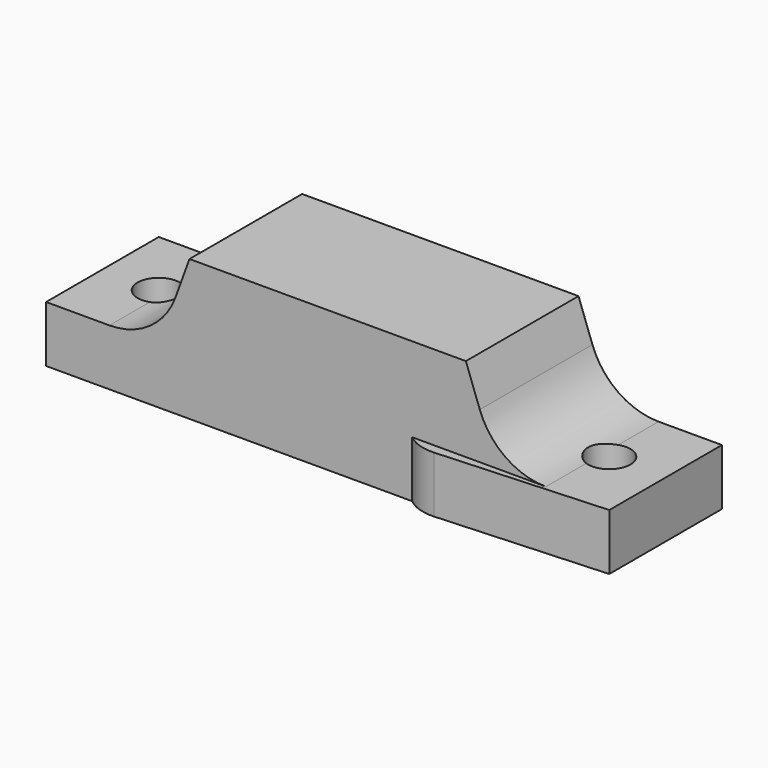
from build123d import *

# Parameters (mm, degrees)
F1_DEPTH    = 5
F2_R        = 5
F3_R        = 1.5
F4_DEPTH    = 25
F6_DEPTH    = 4
F7_T1_DEPTH = 14.4192067173


# Not quite as in the source:
# - a fillet or chamfer that OpenCascade refuses, or shapes differently, is made with other operations: its cross-section is extruded or revolved along the edge and cut away or added


with BuildPart() as f1:
    # F0 (on Front) → F1 (new body, symmetric)
    with BuildSketch(Plane.XZ):
        Polygon((0, 4), (0, 0), (40, 0), (40, 4), (32, 4), (29.8161785944, 10), (10.1838214056, 10), (8, 4), align=None)
    extrude(amount=F1_DEPTH, both=True)

    # F2
    f2_edges = [f1.edges().sort_by_distance(p)[0] for p in [
        (32, 0, 4),
        (8, 0, 4),
    ]]
    fillet(f2_edges, radius=F2_R)

    # F3 (on Top) → F4 (cut)
    with BuildSketch(Plane.XY):
        with Locations((4, 0)):
            Circle(F3_R)
        with Locations((36, 0)):
            Circle(F3_R)
    extrude(amount=F4_DEPTH, mode=Mode.SUBTRACT)

    # F5 (on Top) → F6 (join)
    with BuildSketch(Plane.XY):
        Polygon((26, -5.8), (40, -5), (26, -5), align=None)
    extrude(amount=F6_DEPTH)

    # F7: fillet of radius 3 on 1 edges, made by hand

    # F7_s2 → F7_t1 (cut)
    with BuildSketch(Plane.XY.offset(-5.2096033586)):
        with BuildLine():
            ThreePointArc((26, -5), (26.9758794109, -5.5370959816), (28.0804474628, -5.6811172878))
            Line((28.0804474628, -5.6811172878), (26, -5.8))
            Line((26, -5.8), (26, -5))
        make_face()
    extrude(amount=F7_T1_DEPTH, mode=Mode.SUBTRACT)


solid = f1.part
